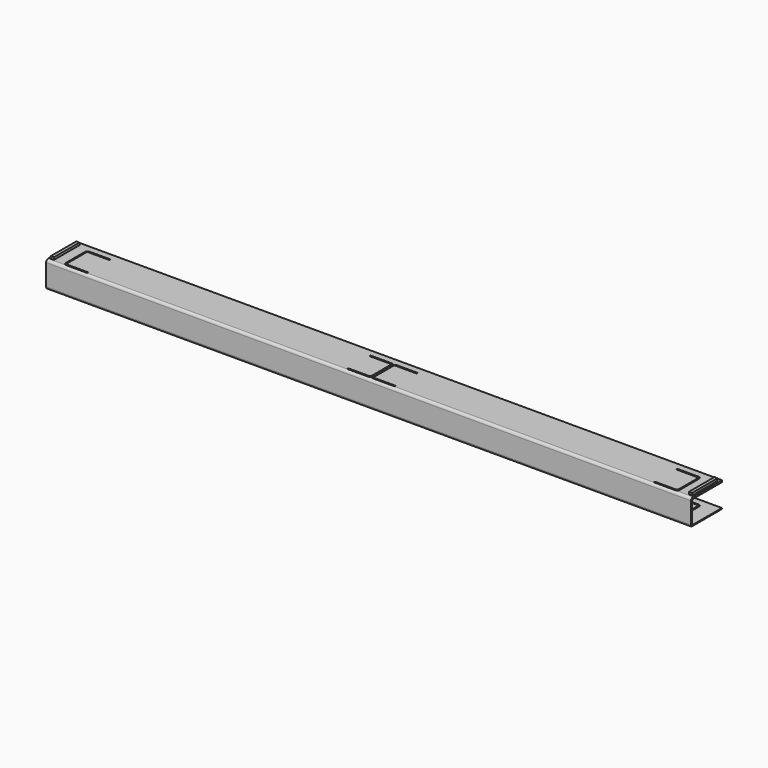
from build123d import *

# Parameters (mm, degrees)
F0_W         = 69
F0_H         = 5.7454954955
F1_DEPTH     = 2050
F2_W         = 10
F2_H         = 101.5
F3_DEPTH     = 7.5
F7_DEPTH     = 84
F10_DEPTH    = 90
F11_T1_DEPTH = 134.5
F12_T1_DEPTH = 139.5


# Not quite as in the source:
# - a fillet or chamfer that OpenCascade refuses, or shapes differently, is made with other operations: its cross-section is extruded or revolved along the edge and cut away or added


with BuildPart() as f1:
    # F0 (on Right) → F1 (new body)
    with BuildSketch(Plane.YZ):
        with BuildLine():
            ThreePointArc((-53.5, -33.75), (-51.1568542495, -39.4068542495), (-45.5, -41.75))
            Line((-45.5, -41.75), (0, -41.75))
            Line((0, -41.75), (0, -36.0045045045))
            Line((0, -36.0045045045), (-45.5, -36.0045045045))
            ThreePointArc((-45.5, -36.0045045045), (-48.3284271247, -34.8329316293), (-49.5, -32.0045045045))
            Line((-49.5, -32.0045045045), (-49.5, 32.0045045045))
            ThreePointArc((-49.5, 32.0045045045), (-48.3284271247, 34.8329316293), (-45.5, 36.0045045045))
            Line((-45.5, 36.0045045045), (0, 36.0045045045))
            Line((0, 36.0045045045), (0, 41.75))
            Line((0, 41.75), (-45.5, 41.75))
            ThreePointArc((-45.5, 41.75), (-51.1568542495, 39.4068542495), (-53.5, 33.75))
            Line((-53.5, 33.75), (-53.5, -33.75))
        make_face()
        with Locations((34.5, 38.8772522523)):
            Rectangle(F0_W, F0_H)
        with Locations((34.5, -38.8772522523)):
            Rectangle(F0_W, F0_H)
    extrude(amount=-F1_DEPTH)

    # F2 (on face) → F3 (join)
    with BuildSketch(Plane.XY.offset(41.75)):
        with Locations((-2039, 8.25)):
            Rectangle(F2_W, F2_H)
    extrude(amount=F3_DEPTH)

    # F5: F1 across plane


with BuildPart() as f1_1:
    add(f1.part)
    add(f1.part.mirror(Plane.YZ.offset(-1025)))

    # F6 (on face) → F7 (cut)
    with BuildSketch(Plane.XY.offset(41.75)):
        with BuildLine():
            Line((-2001, 39.5), (-2001, 0))
            Line((-2001, 0), (-2001, -37.5))
            ThreePointArc((-2001, -37.5), (-1998.6568542495, -43.1568542495), (-1993, -45.5))
            Line((-1993, -45.5), (-1925.5, -45.5))
            Line((-1925.5, -45.5), (-1925.5, -41.25))
            Line((-1925.5, -41.25), (-1984.9698543549, -41.25))
            Line((-1984.9698543549, -41.25), (-1992.75, -41.25))
            ThreePointArc((-1992.75, -41.25), (-1995.5784271247, -40.0784271247), (-1996.75, -37.25))
            Line((-1996.75, -37.25), (-1996.75, 0))
            Line((-1996.75, 0), (-1996.75, 39.25))
            ThreePointArc((-1996.75, 39.25), (-1995.5784271247, 42.0784271247), (-1992.75, 43.25))
            Line((-1992.75, 43.25), (-1925.5, 43.25))
            Line((-1925.5, 43.25), (-1925.5, 47.5))
            Line((-1925.5, 47.5), (-1993, 47.5))
            ThreePointArc((-1993, 47.5), (-1998.6568542495, 45.1568542495), (-2001, 39.5))
        make_face()
    extrude(amount=-F7_DEPTH, mode=Mode.SUBTRACT)

    # F8: F1 across plane


with BuildPart() as f1_2:
    add(f1_1.part)
    add(f1_1.part.mirror(Plane.YZ.offset(-1025)), mode=Mode.INTERSECT)

    # F9 (on face) → F10 (cut)
    with BuildSketch(Plane.XY.offset(41.75)):
        with BuildLine():
            ThreePointArc((-1024.0666470126, -40.75), (-1021.1231056256, -43.8556546004), (-1017, -45))
            Line((-1017, -45), (-950, -45))
            Line((-950, -45), (-950, -40.75))
            Line((-950, -40.75), (-1016.75, -40.75))
            ThreePointArc((-1016.75, -40.75), (-1019.5784271247, -39.5784271247), (-1020.75, -36.75))
            Line((-1020.75, -36.75), (-1020.75, 1.25))
            Line((-1020.75, 1.25), (-1020.75, 39.25))
            ThreePointArc((-1020.75, 39.25), (-1019.5784271247, 42.0784271247), (-1016.75, 43.25))
            Line((-1016.75, 43.25), (-950, 43.25))
            Line((-950, 43.25), (-950, 47.5))
            Line((-950, 47.5), (-1017, 47.5))
            ThreePointArc((-1017, 47.5), (-1021.1231056256, 46.3556546004), (-1024.0666470126, 43.25))
            Line((-1024.0666470126, 43.25), (-1025.9333529874, 43.25))
            ThreePointArc((-1025.9333529874, 43.25), (-1028.8768943744, 46.3556546004), (-1033, 47.5))
            Line((-1033, 47.5), (-1100, 47.5))
            Line((-1100, 47.5), (-1100, 43.25))
            Line((-1100, 43.25), (-1033.25, 43.25))
            ThreePointArc((-1033.25, 43.25), (-1030.4215728753, 42.0784271247), (-1029.25, 39.25))
            Line((-1029.25, 39.25), (-1029.25, 1.25))
            Line((-1029.25, 1.25), (-1029.25, -36.75))
            ThreePointArc((-1029.25, -36.75), (-1030.4215728753, -39.5784271247), (-1033.25, -40.75))
            Line((-1033.25, -40.75), (-1100, -40.75))
            Line((-1100, -40.75), (-1100, -45))
            Line((-1100, -45), (-1033, -45))
            ThreePointArc((-1033, -45), (-1028.8768943744, -43.8556546004), (-1025.9333529874, -40.75))
            Line((-1025.9333529874, -40.75), (-1024.0666470126, -40.75))
        make_face()
    extrude(amount=-F10_DEPTH, mode=Mode.SUBTRACT)

    # F11: fillet of radius 4 on 1 edges, made by hand

    # F11_s2 → F11_t1 (cut)
    with BuildSketch(Plane.XZ.offset(-79)):
        with BuildLine():
            ThreePointArc((-2046, -41.75), (-2048.8284271247, -40.5784271247), (-2050, -37.75))
            Line((-2050, -37.75), (-2050, -41.75))
            Line((-2050, -41.75), (-2046, -41.75))
        make_face()
    extrude(amount=F11_T1_DEPTH, mode=Mode.SUBTRACT)

    # F12: fillet of radius 5 on 1 edges, made by hand

    # F12_s2 → F12_t1 (cut)
    with BuildSketch(Plane.XZ.offset(-81.5)):
        with BuildLine():
            ThreePointArc((0, -36.75), (-1.4644660941, -40.2855339059), (-5, -41.75))
            Line((-5, -41.75), (0, -41.75))
            Line((0, -41.75), (0, -36.75))
        make_face()
    extrude(amount=F12_T1_DEPTH, mode=Mode.SUBTRACT)


solid = f1_2.part
